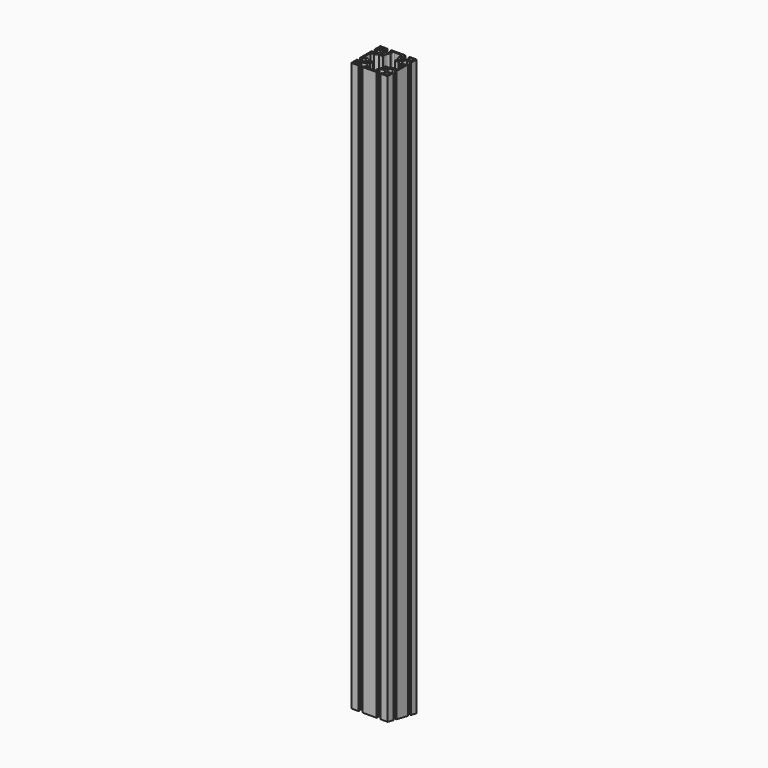
from build123d import *

# Parameters (mm, degrees)
F0_R          = 3
F0_R_2        = 2.5
F1_DEPTH      = 950
F2_R          = 2
F3_R          = 7
F5_DEPTH      = 30
F5_DEPTH_BACK = 30


# Not quite as in the source:
# - a feature names something its author has since deleted; it is built from what else it names


with BuildPart() as f1:
    # F0 (on Top) → F1 (new body)
    with BuildSketch(Plane.XY):
        with BuildLine():
            Line((18.15, -30), (30, -30))
            Line((30, -30), (30, -18.15))
            Line((30, -18.15), (27.5, -18.15))
            Line((27.5, -18.15), (27.5, -20.15))
            Line((27.5, -20.15), (21.5477069044, -20.15))
            ThreePointArc((21.5477069044, -20.15), (19.5, -15), (21.5477069044, -9.85))
            Line((21.5477069044, -9.85), (27.5, -9.85))
            Line((27.5, -9.85), (27.5, -11.85))
            Line((27.5, -11.85), (30, -11.85))
            Line((30, -11.85), (30, 11.85))
            Line((30, 11.85), (27.5, 11.85))
            Line((27.5, 11.85), (27.5, 9.85))
            Line((27.5, 9.85), (21.5477069044, 9.85))
            ThreePointArc((21.5477069044, 9.85), (19.5, 15), (21.5477069044, 20.15))
            Line((21.5477069044, 20.15), (27.5, 20.15))
            Line((27.5, 20.15), (27.5, 18.15))
            Line((27.5, 18.15), (30, 18.15))
            Line((30, 18.15), (30, 30))
            Line((30, 30), (18.15, 30))
            Line((18.15, 30), (18.15, 27.5))
            Line((18.15, 27.5), (20.15, 27.5))
            Line((20.15, 27.5), (20.15, 21.5477069044))
            ThreePointArc((20.15, 21.5477069044), (15, 19.5), (9.85, 21.5477069044))
            Line((9.85, 21.5477069044), (9.85, 27.5))
            Line((9.85, 27.5), (11.85, 27.5))
            Line((11.85, 27.5), (11.85, 30))
            Line((11.85, 30), (-11.85, 30))
            Line((-11.85, 30), (-11.85, 27.5))
            Line((-11.85, 27.5), (-9.85, 27.5))
            Line((-9.85, 27.5), (-9.85, 21.5477069044))
            ThreePointArc((-9.85, 21.5477069044), (-15, 19.5), (-20.15, 21.5477069044))
            Line((-20.15, 21.5477069044), (-20.15, 27.5))
            Line((-20.15, 27.5), (-18.15, 27.5))
            Line((-18.15, 27.5), (-18.15, 30))
            Line((-18.15, 30), (-30, 30))
            Line((-30, 30), (-30, 18.15))
            Line((-30, 18.15), (-27.5, 18.15))
            Line((-27.5, 18.15), (-27.5, 20.15))
            Line((-27.5, 20.15), (-21.5477069044, 20.15))
            ThreePointArc((-21.5477069044, 20.15), (-19.5, 15), (-21.5477069044, 9.85))
            Line((-21.5477069044, 9.85), (-27.5, 9.85))
            Line((-27.5, 9.85), (-27.5, 11.85))
            Line((-27.5, 11.85), (-30, 11.85))
            Line((-30, 11.85), (-30, -11.85))
            Line((-30, -11.85), (-27.5, -11.85))
            Line((-27.5, -11.85), (-27.5, -9.85))
            Line((-27.5, -9.85), (-21.5477069044, -9.85))
            ThreePointArc((-21.5477069044, -9.85), (-19.5, -15), (-21.5477069044, -20.15))
            Line((-21.5477069044, -20.15), (-27.5, -20.15))
            Line((-27.5, -20.15), (-27.5, -18.15))
            Line((-27.5, -18.15), (-30, -18.15))
            Line((-30, -18.15), (-30, -30))
            Line((-30, -30), (-18.15, -30))
            Line((-18.15, -30), (-18.15, -27.5))
            Line((-18.15, -27.5), (-20.15, -27.5))
            Line((-20.15, -27.5), (-20.15, -21.5477069044))
            ThreePointArc((-20.15, -21.5477069044), (-15, -19.5), (-9.85, -21.5477069044))
            Line((-9.85, -21.5477069044), (-9.85, -27.5))
            Line((-9.85, -27.5), (-11.85, -27.5))
            Line((-11.85, -27.5), (-11.85, -30))
            Line((-11.85, -30), (11.85, -30))
            Line((11.85, -30), (11.85, -27.5))
            Line((11.85, -27.5), (9.85, -27.5))
            Line((9.85, -27.5), (9.85, -21.5477069044))
            ThreePointArc((9.85, -21.5477069044), (15, -19.5), (20.15, -21.5477069044))
            Line((20.15, -21.5477069044), (20.15, -27.5))
            Line((20.15, -27.5), (18.15, -27.5))
            Line((18.15, -27.5), (18.15, -30))
        make_face()
        with Locations((-25, -25)):
            Circle(F0_R, mode=Mode.SUBTRACT)
        with Locations((-15, -15)):
            Circle(F0_R_2, mode=Mode.SUBTRACT)
        with Locations((25, -25)):
            Circle(F0_R, mode=Mode.SUBTRACT)
        with Locations((15, -15)):
            Circle(F0_R_2, mode=Mode.SUBTRACT)
        with Locations((-25, 25)):
            Circle(F0_R, mode=Mode.SUBTRACT)
        with Locations((-15, 15)):
            Circle(F0_R_2, mode=Mode.SUBTRACT)
        Polygon((-7, 22), (-7, 27.5), (0, 27.5), (7, 27.5), (7, 22), (10, 16), (10, 10), (16, 10), (22, 7), (27.5, 7), (27.5, 0), (27.5, -7), (22, -7), (16, -10), (10, -10), (10, -16), (7, -22), (7, -27.5), (0, -27.5), (-7, -27.5), (-7, -22), (-10, -16), (-10, -10), (-16, -10), (-22, -7), (-27.5, -7), (-27.5, 0), (-27.5, 7), (-22, 7), (-16, 10), (-10, 10), (-10, 16), align=None, mode=Mode.SUBTRACT)
        with Locations((15, 15)):
            Circle(F0_R_2, mode=Mode.SUBTRACT)
        with Locations((25, 25)):
            Circle(F0_R, mode=Mode.SUBTRACT)
    extrude(amount=F1_DEPTH)

    # F2
    f2_edges = [f1.edges().sort_by_distance(p)[0] for p in [
        (-7, 27.5, 475),
        (7, 27.5, 475),
    ]]
    fillet(f2_edges, radius=F2_R)

    # F3
    f3_edges = [f1.edges().sort_by_distance(p)[0] for p in [
        (-10, 16, 475),
        (10, 16, 475),
    ]]
    fillet(f3_edges, radius=F3_R)

    # F4 (on Right) → F5 (cut, two sides)
    with BuildSketch(Plane.YZ) as f5_sk:
        Polygon((-164.2855995683, 38.6458085579), (-188.5911429791, -83.5464097089), (5.6944565892, -122.1922182668), (30, 0), align=None)
    extrude(amount=F5_DEPTH, mode=Mode.SUBTRACT)
    extrude(f5_sk.sketch, amount=-F5_DEPTH_BACK, mode=Mode.SUBTRACT)


solid = f1.part
